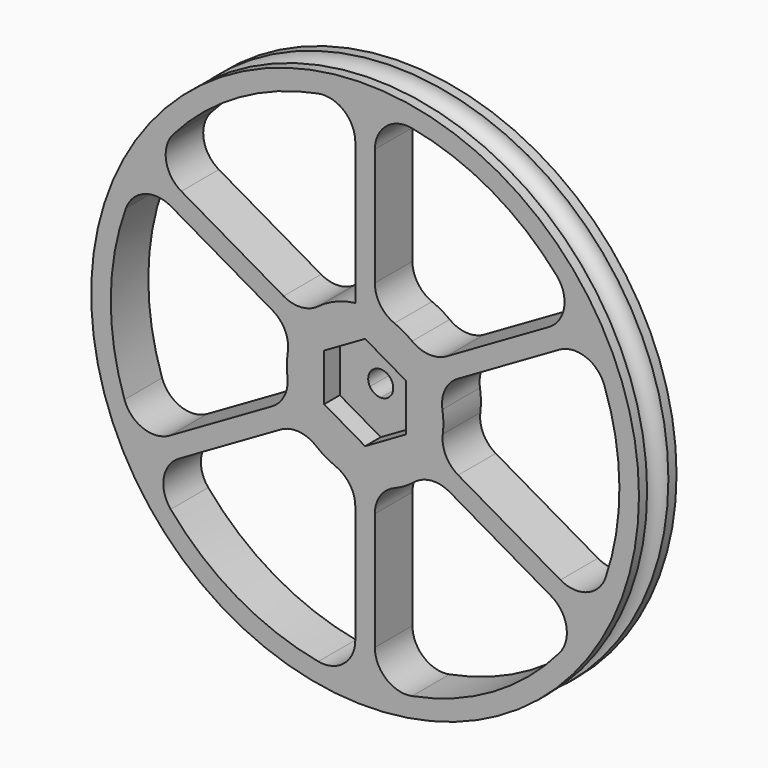
from build123d import *

# Parameters (mm, degrees)
F0_W      = 44.45
F0_H      = 1.651
F2_R      = 41.275
F3_DEPTH  = 7.621
F5_DEPTH  = 3.81
F6_DEPTH  = 3.81
F7_DEPTH  = 3.81
F9_DEPTH  = 3.175
F10_DEPTH = 7.621
F11_R     = 5.08


# Not quite as in the source:
# - two fillets or chamfers of one size are made in one step
# - ends of sketch curves that miss each other by under 0.0002 mm in the source are joined
# - a feature names something its author has since deleted; it is built from what else it names


with BuildPart() as f1:
    # F0 (on Top) → F1 (revolve)
    with BuildSketch(Plane.XY):
        with Locations((22.225, 2.9845)):
            Rectangle(F0_W, F0_H)
        with Locations((22.225, -2.9845)):
            Rectangle(F0_W, F0_H)
        with BuildLine():
            Line((0, 2.159), (0, 0))
            Line((0, 0), (0, -2.159))
            Line((0, -2.159), (44.45, -2.159))
            ThreePointArc((44.45, -2.159), (42.291, 0), (44.45, 2.159))
            Line((44.45, 2.159), (0, 2.159))
        make_face()
    revolve(axis=Axis((0, -1.905, 0), (0, -1, 0)))

    # F2 (on face) → F3 (cut, through all)
    with BuildSketch(Plane(origin=(0, 3.81, 0), x_dir=(-1, 0, 0), z_dir=(0, 1, 0))):
        Circle(F2_R)
    extrude(amount=-F3_DEPTH, mode=Mode.SUBTRACT)

    # F4 (on Front) → F5 (join, symmetric)
    with BuildSketch(Plane.XZ):
        with BuildLine():
            ThreePointArc((9.9410923172, 7.9034602258), (10.4172850275, 7.2643081333), (10.85244705, 6.5965440214))
            Line((10.85244705, 6.5965440214), (35.8685432444, 21.0395938934))
            ThreePointArc((35.8685432444, 21.0395938934), (35.4602658033, 21.72064582), (35.0390585298, 22.3937777747))
            Line((35.0390585298, 22.3937777747), (9.9410923172, 7.9034602258))
        make_face()
        with BuildLine():
            Line((35.8685432444, 21.0395938934), (10.85244705, 6.5965440214))
            ThreePointArc((10.85244705, 6.5965440214), (11.2438105409, 5.9048052059), (11.5911393429, 5.1899411109))
            Line((11.5911393429, 5.1899411109), (36.6455202991, 19.6550947004))
            ThreePointArc((36.6455202991, 19.6550947004), (36.263639674, 20.351052633), (35.8685432444, 21.0395938934))
        make_face()
        with BuildLine():
            Line((0, 41.583853906), (0, 12.7))
            ThreePointArc((0, 12.7), (0.7953109893, 12.6750731923), (1.5875, 12.6003906189))
            Line((1.5875, 12.6003906189), (1.5875, 41.5535407568))
            ThreePointArc((1.5875, 41.5535407568), (0.7938946934, 41.576274928), (0, 41.583853906))
        make_face()
        with BuildLine():
            ThreePointArc((-1.5875, 12.6003906189), (-0.7953109893, 12.6750731923), (0, 12.7))
            Line((0, 12.7), (0, 41.583853906))
            ThreePointArc((0, 41.583853906), (-0.7938946934, 41.576274928), (-1.5875, 41.5535407568))
            Line((-1.5875, 41.5535407568), (-1.5875, 12.6003906189))
        make_face()
        with BuildLine():
            Line((-35.8685432444, 21.0395938934), (-10.85244705, 6.5965440214))
            ThreePointArc((-10.85244705, 6.5965440214), (-10.4172850275, 7.2643081333), (-9.9410923172, 7.9034602258))
            Line((-9.9410923172, 7.9034602258), (-35.0390585298, 22.3937777747))
            ThreePointArc((-35.0390585298, 22.3937777747), (-35.4602658033, 21.72064582), (-35.8685432444, 21.0395938934))
        make_face()
        with BuildLine():
            ThreePointArc((-11.5911393429, 5.1899411109), (-11.2438105409, 5.9048052059), (-10.85244705, 6.5965440214))
            Line((-10.85244705, 6.5965440214), (-35.8685432444, 21.0395938934))
            ThreePointArc((-35.8685432444, 21.0395938934), (-36.263639674, 20.351052633), (-36.6455202991, 19.6550947004))
            Line((-36.6455202991, 19.6550947004), (-11.5911393429, 5.1899411109))
        make_face()
        with BuildLine():
            Line((-36.1550944192, -20.5432726997), (-11.1389982248, -6.1002228278))
            ThreePointArc((-11.1389982248, -6.1002228278), (-11.4997178981, -5.3894794057), (-11.8151434919, -4.6575083752))
            Line((-11.8151434919, -4.6575083752), (-36.9131097045, -19.1478259241))
            ThreePointArc((-36.9131097045, -19.1478259241), (-36.5407639684, -19.8491681006), (-36.1550944192, -20.5432726997))
        make_face()
        with BuildLine():
            ThreePointArc((-10.2901905176, -7.4432505743), (-10.7356165832, -6.7850229608), (-11.1389982248, -6.1002228278))
            Line((-11.1389982248, -6.1002228278), (-36.1550944192, -20.5432726997))
            ThreePointArc((-36.1550944192, -20.5432726997), (-35.7563484109, -21.2297068748), (-35.3445714739, -21.9084041638))
            Line((-35.3445714739, -21.9084041638), (-10.2901905176, -7.4432505743))
        make_face()
        with BuildLine():
            Line((36.1550944192, -20.5432726997), (11.1389982248, -6.1002228278))
            ThreePointArc((11.1389982248, -6.1002228278), (10.7356165832, -6.7850229608), (10.2901905176, -7.4432505743))
            Line((10.2901905176, -7.4432505743), (35.3445714739, -21.9084041638))
            ThreePointArc((35.3445714739, -21.9084041638), (35.7563484109, -21.2297068748), (36.1550944192, -20.5432726997))
        make_face()
        with BuildLine():
            ThreePointArc((11.8151434743, -4.6575084199), (11.4997178879, -5.3894794275), (11.1389982248, -6.1002228278))
            Line((11.1389982248, -6.1002228278), (36.1550944192, -20.5432726997))
            ThreePointArc((36.1550944192, -20.5432726997), (36.5407639684, -19.8491681006), (36.9131097045, -19.1478259241))
            Line((36.9131097045, -19.1478259241), (11.8151434743, -4.6575084199))
        make_face()
        with BuildLine():
            ThreePointArc((1.5875, -12.6003906189), (0.7953109893, -12.6750731923), (0, -12.7))
            Line((0, -12.7), (0, -41.583853906))
            ThreePointArc((0, -41.583853906), (0.7938946934, -41.576274928), (1.5875, -41.5535407568))
            Line((1.5875, -41.5535407568), (1.5875, -12.6003906189))
        make_face()
        with BuildLine():
            Line((0, -41.583853906), (0, -12.7))
            ThreePointArc((0, -12.7), (-0.7953109893, -12.6750731923), (-1.5875, -12.6003906189))
            Line((-1.5875, -12.6003906189), (-1.5875, -41.5535407568))
            ThreePointArc((-1.5875, -41.5535407568), (-0.7938946934, -41.576274928), (0, -41.583853906))
        make_face()
    extrude(amount=F5_DEPTH, both=True)

    # F4 (on Front) → F6 (join, symmetric)
    with BuildSketch(Plane.XZ):
        with BuildLine():
            Line((10.85244705, 6.5965440214), (8.3535925717, 5.1538297157))
            ThreePointArc((8.3535925717, 5.1538297157), (9.4429693471, 2.6785816216), (9.8155218706, 0))
            ThreePointArc((9.8155218706, 0), (9.5171421524, -2.4017649436), (8.640143746, -4.6575085229))
            Line((8.6401437743, -4.6575085382), (11.1389982248, -6.1002228278))
            ThreePointArc((11.1389982248, -6.1002228278), (11.4997178879, -5.3894794275), (11.8151434743, -4.6575084199))
            ThreePointArc((11.8151434743, -4.6575084199), (12.4768249592, -2.3704090234), (12.7, 0))
            ThreePointArc((12.7, 0), (12.4196914143, 2.6535382366), (11.5911393429, 5.1899411109))
            ThreePointArc((11.5911393429, 5.1899411109), (11.2438105409, 5.9048052059), (10.85244705, 6.5965440214))
        make_face()
        with BuildLine():
            Line((0, 12.7), (0, 9.8155218706))
            ThreePointArc((0, 9.8155218706), (4.7831444313, 8.5712308884), (8.3535925717, 5.1538297157))
            Line((8.3535925717, 5.1538297157), (10.85244705, 6.5965440214))
            ThreePointArc((10.85244705, 6.5965440214), (10.4172850275, 7.2643081333), (9.9410923172, 7.9034602258))
            ThreePointArc((9.9410923172, 7.9034602258), (6.2243392407, 11.0701219965), (1.5875, 12.6003906189))
            ThreePointArc((1.5875, 12.6003906189), (0.7953109893, 12.6750731923), (0, 12.7))
        make_face()
        with BuildLine():
            Line((-10.85244705, 6.5965440214), (-8.3535925717, 5.1538297157))
            ThreePointArc((-8.3535925717, 5.1538297157), (-4.7831444313, 8.5712308884), (0, 9.8155218706))
            Line((0, 9.8155218706), (0, 12.7))
            ThreePointArc((0, 12.7), (-0.7953109893, 12.6750731923), (-1.5875, 12.6003906189))
            ThreePointArc((-1.5875, 12.6003906189), (-6.2243392407, 11.0701219965), (-9.9410923172, 7.9034602258))
            ThreePointArc((-9.9410923172, 7.9034602258), (-10.4172850275, 7.2643081333), (-10.85244705, 6.5965440214))
        make_face()
        with BuildLine():
            ThreePointArc((-8.6401437465, -4.6575085221), (-9.8113382378, 0.2865511747), (-8.3535925717, 5.1538297157))
            Line((-8.3535925717, 5.1538297157), (-10.85244705, 6.5965440214))
            ThreePointArc((-10.85244705, 6.5965440214), (-11.2438105409, 5.9048052059), (-11.5911393429, 5.1899411109))
            ThreePointArc((-11.5911393429, 5.1899411109), (-12.6967154958, 0.2888176228), (-11.8151434919, -4.6575083752))
            ThreePointArc((-11.8151434919, -4.6575083752), (-11.4997178981, -5.3894794057), (-11.1389982248, -6.1002228278))
            Line((-11.1389982248, -6.1002228278), (-8.6401437465, -4.6575085221))
        make_face()
        with BuildLine():
            ThreePointArc((0, -9.8155218706), (-5.0313314754, -8.4279400316), (-8.6401437465, -4.6575085221))
            Line((-8.6401437465, -4.6575085221), (-11.1389982248, -6.1002228278))
            ThreePointArc((-11.1389982248, -6.1002228278), (-10.7356165832, -6.7850229608), (-10.2901905176, -7.4432505743))
            ThreePointArc((-10.2901905176, -7.4432505743), (-6.4744811659, -10.9257079236), (-1.5875, -12.6003906189))
            ThreePointArc((-1.5875, -12.6003906189), (-0.7953109893, -12.6750731923), (0, -12.7))
            Line((0, -12.7), (0, -9.8155218706))
        make_face()
        with BuildLine():
            ThreePointArc((8.640143746, -4.6575085229), (5.031331475, -8.4279400319), (0, -9.8155218706))
            Line((0, -9.8155218706), (0, -12.7))
            ThreePointArc((0, -12.7), (0.7953109893, -12.6750731923), (1.5875, -12.6003906189))
            ThreePointArc((1.5875, -12.6003906189), (6.4744811659, -10.9257079236), (10.2901905176, -7.4432505743))
            ThreePointArc((10.2901905176, -7.4432505743), (10.7356165832, -6.7850229608), (11.1389982248, -6.1002228278))
            Line((11.1389982248, -6.1002228278), (8.6401437743, -4.6575085382))
        make_face()
        with BuildLine():
            Line((8.3535925717, 5.1538297157), (6.6421, 4.1656990187))
            Line((6.6421, 4.1656990187), (6.6421, -3.5039374272))
            Line((6.6421, -3.5039374272), (8.6401437743, -4.6575085382))
            ThreePointArc((8.640143746, -4.6575085229), (9.5171421524, -2.4017649436), (9.8155218706, 0))
            ThreePointArc((9.8155218706, 0), (9.4429693471, 2.6785816216), (8.3535925717, 5.1538297157))
        make_face()
        with BuildLine():
            Line((6.6421, -3.5039374272), (0, -7.3387556502))
            Line((0, -7.3387556502), (0, -9.8155218706))
            ThreePointArc((0, -9.8155218706), (5.031331475, -8.4279400319), (8.640143746, -4.6575085229))
            Line((8.6401437743, -4.6575085382), (6.6421, -3.5039374272))
        make_face()
        with BuildLine():
            Line((0, -7.3387556502), (-6.6421, -3.5039374272))
            Line((-6.6421, -3.5039374272), (-8.6401437465, -4.6575085221))
            ThreePointArc((-8.6401437465, -4.6575085221), (-5.0313314754, -8.4279400316), (0, -9.8155218706))
            Line((0, -9.8155218706), (0, -7.3387556502))
        make_face()
        with BuildLine():
            Line((-6.6421, -3.5039374272), (-6.6421, 4.1656990187))
            Line((-6.6421, 4.1656990187), (-8.3535925717, 5.1538297157))
            ThreePointArc((-8.3535925717, 5.1538297157), (-9.8113382378, 0.2865511747), (-8.6401437465, -4.6575085221))
            Line((-8.6401437465, -4.6575085221), (-6.6421, -3.5039374272))
        make_face()
        with BuildLine():
            Line((-8.3535925717, 5.1538297157), (-6.6421, 4.1656990187))
            Line((-6.6421, 4.1656990187), (0, 8.0005172417))
            Line((0, 8.0005172417), (0, 9.8155218706))
            ThreePointArc((0, 9.8155218706), (-4.7831444313, 8.5712308884), (-8.3535925717, 5.1538297157))
        make_face()
        with BuildLine():
            Line((0, 9.8155218706), (0, 8.0005172417))
            Line((0, 8.0005172417), (6.6421, 4.1656990187))
            Line((6.6421, 4.1656990187), (8.3535925717, 5.1538297157))
            ThreePointArc((8.3535925717, 5.1538297157), (4.7831444313, 8.5712308884), (0, 9.8155218706))
        make_face()
    extrude(amount=F6_DEPTH, both=True)

    # F4 (on Front) → F7 (join, symmetric)
    with BuildSketch(Plane.XZ):
        Polygon((0, 0.3308807958), (-6.6421, -3.5039374272), (0, -7.3387556502), align=None)
        Polygon((0, 0.3308807958), (-6.6421, 4.1656990187), (-6.6421, -3.5039374272), align=None)
        Polygon((0, 8.0005172417), (-6.6421, 4.1656990187), (0, 0.3308807958), align=None)
        Polygon((6.6421, 4.1656990187), (0, 8.0005172417), (0, 0.3308807958), align=None)
        Polygon((6.6421, 4.1656990187), (0, 0.3308807958), (6.6421, -3.5039374272), align=None)
        Polygon((6.6421, -3.5039374272), (0, 0.3308807958), (0, -7.3387556502), align=None)
    extrude(amount=F7_DEPTH, both=True)

    # F8 (on face) → F9 (cut)
    with BuildSketch(Plane.XZ.offset(3.81)):
        with BuildLine():
            Line((6.6421, -3.5039374272), (6.6421, 4.1656990187))
            Line((6.6421, 4.1656990187), (1.7597636205, 1.3468807958))
            ThreePointArc((1.7597636205, 1.3468807958), (1.962761279, 0.8568010954), (2.032, 0.3308807958))
            ThreePointArc((2.032, 0.3308807958), (1.962761279, -0.1950395039), (1.7597636205, -0.6851192042))
            Line((1.7597636205, -0.6851192042), (6.6421, -3.5039374272))
        make_face()
        with BuildLine():
            Line((0, -1.7011192042), (0, -7.3387556502))
            Line((0, -7.3387556502), (6.6421, -3.5039374272))
            Line((6.6421, -3.5039374272), (1.7597636205, -0.6851192042))
            ThreePointArc((1.7597636205, -0.6851192042), (1.016, -1.4288828247), (0, -1.7011192042))
        make_face()
        with BuildLine():
            Line((-1.7597636205, -0.6851192042), (-6.6421, -3.5039374272))
            Line((-6.6421, -3.5039374272), (0, -7.3387556502))
            Line((0, -7.3387556502), (0, -1.7011192042))
            ThreePointArc((0, -1.7011192042), (-1.016, -1.4288828247), (-1.7597636205, -0.6851192042))
        make_face()
        with BuildLine():
            Line((-1.7597636205, 1.3468807958), (-6.6421, 4.1656990187))
            Line((-6.6421, 4.1656990187), (-6.6421, -3.5039374272))
            Line((-6.6421, -3.5039374272), (-1.7597636205, -0.6851192042))
            ThreePointArc((-1.7597636205, -0.6851192042), (-2.032, 0.3308807958), (-1.7597636205, 1.3468807958))
        make_face()
        with BuildLine():
            Line((0, 8.0005172417), (-6.6421, 4.1656990187))
            Line((-6.6421, 4.1656990187), (-1.7597636205, 1.3468807958))
            ThreePointArc((-1.7597636205, 1.3468807958), (-1.016, 2.0906444162), (0, 2.3628807958))
            Line((0, 2.3628807958), (0, 8.0005172417))
        make_face()
        with BuildLine():
            Line((6.6421, 4.1656990187), (0, 8.0005172417))
            Line((0, 8.0005172417), (0, 2.3628807958))
            ThreePointArc((0, 2.3628807958), (1.016, 2.0906444162), (1.7597636205, 1.3468807958))
            Line((1.7597636205, 1.3468807958), (6.6421, 4.1656990187))
        make_face()
    extrude(amount=-F9_DEPTH, mode=Mode.SUBTRACT)

    # F8 (on face) → F10 (cut, through all)
    with BuildSketch(Plane.XZ.offset(3.81)):
        with BuildLine():
            Line((0, -1.7011192042), (0, 0.3308807958))
            Line((0, 0.3308807958), (-1.7597636205, -0.6851192042))
            ThreePointArc((-1.7597636205, -0.6851192042), (-1.016, -1.4288828247), (0, -1.7011192042))
        make_face()
        with BuildLine():
            Line((0, 0.3308807958), (-1.7597636205, 1.3468807958))
            ThreePointArc((-1.7597636205, 1.3468807958), (-2.032, 0.3308807958), (-1.7597636205, -0.6851192042))
            Line((-1.7597636205, -0.6851192042), (0, 0.3308807958))
        make_face()
        with BuildLine():
            ThreePointArc((0, 2.3628807958), (-1.016, 2.0906444162), (-1.7597636205, 1.3468807958))
            Line((-1.7597636205, 1.3468807958), (0, 0.3308807958))
            Line((0, 0.3308807958), (0, 2.3628807958))
        make_face()
        with BuildLine():
            ThreePointArc((1.7597636205, 1.3468807958), (1.016, 2.0906444162), (0, 2.3628807958))
            Line((0, 2.3628807958), (0, 0.3308807958))
            Line((0, 0.3308807958), (1.7597636205, 1.3468807958))
        make_face()
        with BuildLine():
            Line((1.7597636205, 1.3468807958), (0, 0.3308807958))
            Line((0, 0.3308807958), (1.7597636205, -0.6851192042))
            ThreePointArc((1.7597636205, -0.6851192042), (1.962761279, -0.1950395039), (2.032, 0.3308807958))
            ThreePointArc((2.032, 0.3308807958), (1.962761279, 0.8568010954), (1.7597636205, 1.3468807958))
        make_face()
        with BuildLine():
            Line((1.7597636205, -0.6851192042), (0, 0.3308807958))
            Line((0, 0.3308807958), (0, -1.7011192042))
            ThreePointArc((0, -1.7011192042), (1.016, -1.4288828247), (1.7597636205, -0.6851192042))
        make_face()
    extrude(amount=-F10_DEPTH, mode=Mode.SUBTRACT)

    # F11
    f11_edges = [f1.edges().sort_by_distance(p)[0] for p in [
        (1.5875, 0, -41.24446),
        (-1.5875, 0, -41.24446),
        (36.64536, 0, -18.993241),
        (35.076964, 0, -21.753901),
        (34.771309, 0, 22.239193),
        (36.377913, 0, 19.500592),
        (-1.5875, 0, 41.24446),
        (-9.941092, 0, 7.90346),
        (-34.771309, 0, 22.239193),
        (-11.591139, 0, 5.189941),
        (-11.815143, 0, -4.657508),
        (-36.377913, 0, 19.500592),
        (-36.64536, 0, -18.993241),
        (1.5875, 0, 12.600391),
        (1.5875, 0, 41.24446),
        (9.941092, 0, 7.90346),
        (11.591139, 0, 5.189941),
        (11.815143, 0, -4.657508),
        (-1.5875, 0, -12.600391),
        (-10.290191, 0, -7.443251),
        (-35.076964, 0, -21.753901),
        (10.290191, 0, -7.443251),
        (1.5875, 0, -12.600391),
    ]]
    fillet(f11_edges, radius=F11_R)


solid = f1.part
